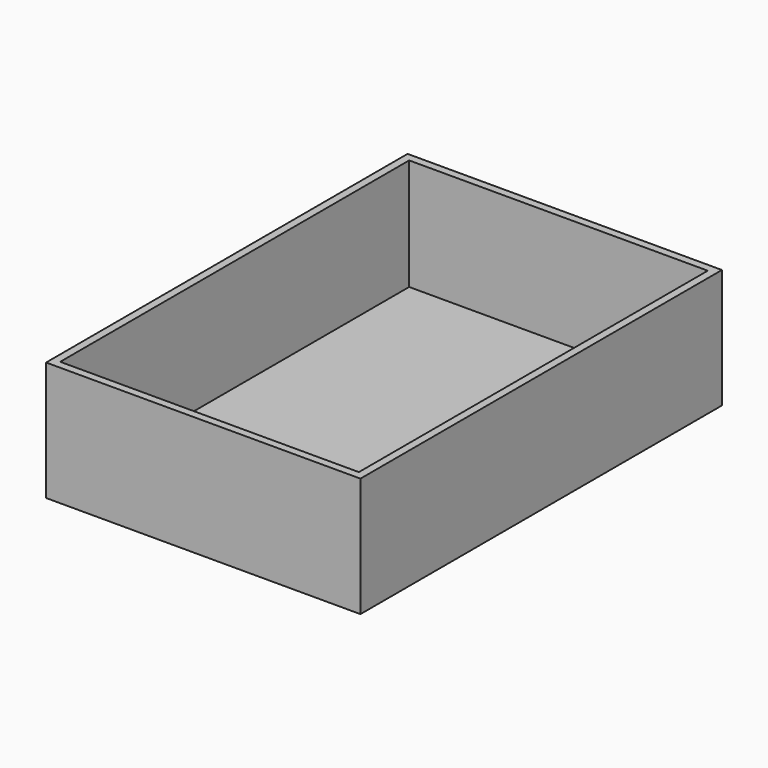
from build123d import *

# Parameters (mm, degrees)
F0_W     = 101.6
F0_H     = 146.05
F1_DEPTH = 25.4
F2_T     = -2.54
F3_DEPTH = 13.157164678


with BuildPart() as f1:
    # F0 (on Top) → F1 (new body)
    with BuildSketch(Plane.XY):
        with Locations((-8.3804931492, -9.2198206152)):
            Rectangle(F0_W, F0_H)
    extrude(amount=F1_DEPTH)

    # F2
    f2_openings = [f1.faces().sort_by_distance(p)[0] for p in [
        (-8.380493, -9.219821, 25.4),
    ]]
    offset(amount=F2_T, openings=f2_openings)

    # F3 (add): a face of the model
    f3_faces = [f1.faces().sort_by_distance(p)[0] for p in [
        (40.6403732836, -9.2198206152, 25.4),
    ]]
    extrude(f3_faces, amount=F3_DEPTH)


solid = f1.part
